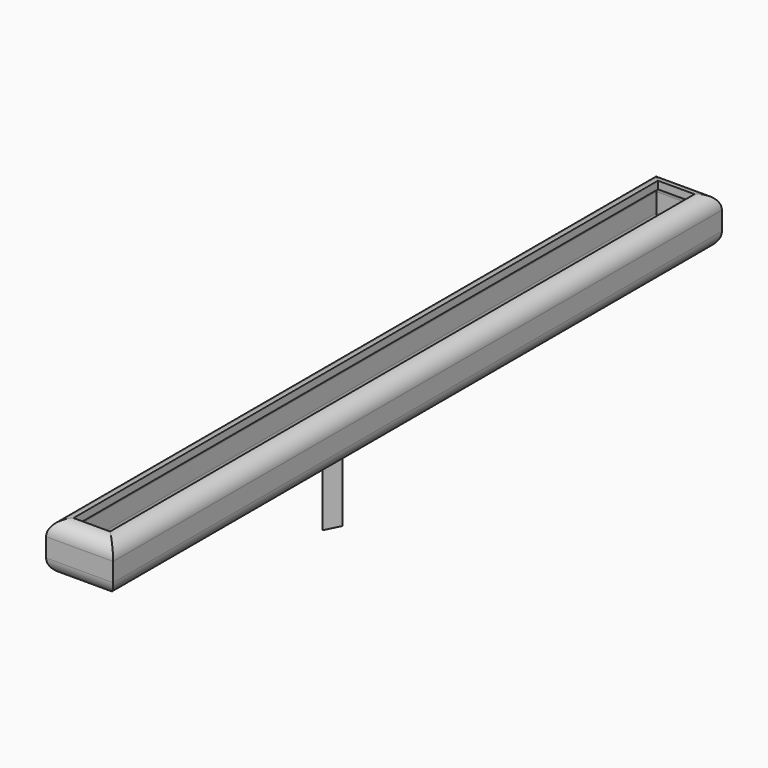
from build123d import *

# Parameters (mm, degrees)
F0_W           = 22.3758686334
F0_H           = 16.4037477225
F1_DEPTH       = 254
F2_R           = 5.08
F3_T           = -2.54
F5_DEPTH       = 25.4
F7_D           = 5.5
F7_CSINK_D     = 11.2
F7_CSINK_ANGLE = 90


# Not quite as in the source:
# - a shell that OpenCascade refuses in one call is made with other operations: the cavity is built on its own and cut out


with BuildPart() as f1:
    # F0 (on Front) → F1 (new body)
    with BuildSketch(Plane.XZ):
        with Locations((-11.1879343167, -8.2018738613)):
            Rectangle(F0_W, F0_H)
    extrude(amount=F1_DEPTH)

    # F2
    f2_edges = [f1.edges().sort_by_distance(p)[0] for p in [
        (0, -127, 0),
        (-22.375869, -127, 0),
        (-11.187934, 0, 0),
        (-11.187934, -254, 0),
        (-22.375869, -127, -16.403748),
        (0, -127, -16.403748),
        (-11.187934, 0, -16.403748),
        (-11.187934, -254, -16.403748),
    ]]
    fillet(f2_edges, radius=F2_R)

    # F3: a shell. OpenCascade refuses it in one call, so the cavity is built on its own and cut out:
    # the body offset inwards by the wall thickness, plus a prism from it out through each open face.
    f3_core = offset(f1.part, amount=F3_T, mode=Mode.PRIVATE)
    f3_exits = [f3_core.faces().sort_by_distance(p)[0] for p in [
        (-11.187934, -127, -2.54),
    ]]
    add(f3_core, mode=Mode.SUBTRACT)
    extrude(f3_exits, amount=-F3_T, mode=Mode.SUBTRACT)

    # F4 (on face) → F5 (join)
    with BuildSketch(Plane(origin=(0, 0, -16.4037477225), x_dir=(1, 0, 0), z_dir=(0, 0, -1))):
        Polygon((-14.9793126683, 145.9724638483), (-12.4393126683, 145.9724638483), (-9.8993126683, 145.9724638483), (-12.4393126683, 151.0524716356), align=None)
    extrude(amount=F5_DEPTH)

    # F7 (through all)
    with Locations(Plane(origin=(0, 0, -16.4037477225), x_dir=(1, 0, 0), z_dir=(0, 0, -1))):
        with Locations((-10.6817428023, 79.9587219954)):
            CounterSinkHole(F7_D / 2, F7_CSINK_D / 2, counter_sink_angle=F7_CSINK_ANGLE)


solid = f1.part
